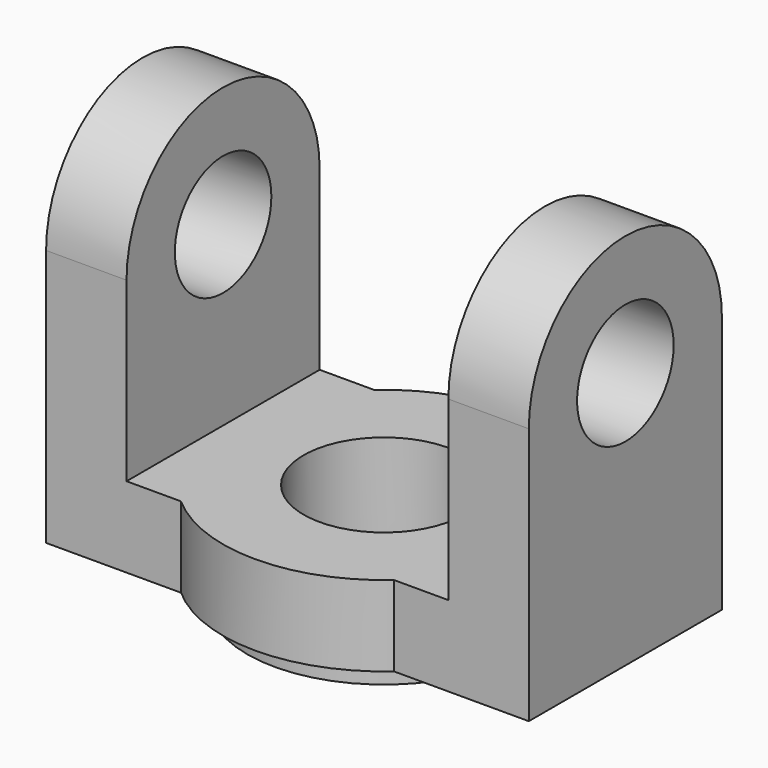
from build123d import *

# Parameters (mm, degrees)
F0_W      = 60
F0_H      = 10
F1_DEPTH  = 30
F3_DEPTH  = 3
F5_DEPTH  = 10
F6_R      = 10
F7_DEPTH  = 25
F8_R      = 10
F9_DEPTH  = 3
F10_W     = 10
F10_H     = 30
F11_DEPTH = 22
F12_R     = 15
F13_DEPTH = 10
F14_R     = 15
F15_DEPTH = 10
F16_R     = 7.5
F17_DEPTH = 60


with BuildPart() as f1:
    # F0 (on Front) → F1 (new body)
    with BuildSketch(Plane.XZ):
        with Locations((30, 5)):
            Rectangle(F0_W, F0_H)
    extrude(amount=F1_DEPTH)

    # F2 (on face) → F3 (join)
    with BuildSketch(Plane(origin=(0, 0, 0), x_dir=(1, 0, 0), z_dir=(0, 0, -1))):
        with BuildLine():
            ThreePointArc((22, 30), (13, 15), (22, 0))
            Line((22, 0), (38, 0))
            ThreePointArc((38, 0), (44.5773797371, 6.2535721577), (47, 15))
            ThreePointArc((47, 15), (44.5773797371, 23.7464278423), (38, 30))
            Line((38, 30), (22, 30))
        make_face()
        with BuildLine():
            ThreePointArc((38, 30), (30, 32), (22, 30))
            Line((22, 30), (38, 30))
        make_face()
    extrude(amount=F3_DEPTH)

    # F4 (on face) → F5 (join)
    with BuildSketch(Plane.XY.offset(10)):
        with BuildLine():
            ThreePointArc((43.2287565553, -30), (48.2287565553, -23.2287565553), (50, -15))
            ThreePointArc((50, -15), (48.2287565553, -6.7712434447), (43.2287565553, 0))
            Line((43.2287565553, 0), (16.7712434447, 0))
            ThreePointArc((16.7712434447, 0), (10, -15), (16.7712434447, -30))
            Line((16.7712434447, -30), (43.2287565553, -30))
        make_face()
        with BuildLine():
            Line((16.7712434447, 0), (43.2287565553, 0))
            ThreePointArc((43.2287565553, 0), (30, 5), (16.7712434447, 0))
        make_face()
        with BuildLine():
            ThreePointArc((16.7712434447, -30), (30, -35), (43.2287565553, -30))
            Line((43.2287565553, -30), (16.7712434447, -30))
        make_face()
    extrude(amount=-F5_DEPTH)

    # F6 (on face) → F7 (cut)
    with BuildSketch(Plane.XY.offset(10)):
        with Locations((30, -15)):
            Circle(F6_R)
    extrude(amount=-F7_DEPTH, mode=Mode.SUBTRACT)

    # F8 (on face) → F9 (join)
    with BuildSketch(Plane(origin=(0, 0, -3), x_dir=(1, 0, 0), z_dir=(0, 0, -1))):
        with BuildLine():
            ThreePointArc((38, 0), (44.5773797371, 6.2535721577), (47, 15))
            ThreePointArc((47, 15), (44.5773797371, 23.7464278423), (38, 30))
            Line((38, 30), (22, 30))
            ThreePointArc((22, 30), (13, 15), (22, 0))
            Line((22, 0), (38, 0))
        make_face()
        with Locations((30, 15)):
            Circle(F8_R, mode=Mode.SUBTRACT)
        with BuildLine():
            ThreePointArc((22, 0), (30, -2), (38, 0))
            Line((38, 0), (22, 0))
        make_face()
    extrude(amount=-F9_DEPTH)

    # F10 (on face) → F11 (join)
    with BuildSketch(Plane.XY.offset(10)):
        with Locations((5, -15)):
            Rectangle(F10_W, F10_H)
        with Locations((55, -15)):
            Rectangle(F10_W, F10_H)
    extrude(amount=F11_DEPTH)

    # F12 (on face) → F13 (join)
    with BuildSketch(Plane(origin=(0, 0, 0), x_dir=(0, -1, 0), z_dir=(-1, 0, 0))):
        with Locations((15, 32)):
            Circle(F12_R)
    extrude(amount=-F13_DEPTH)

    # F14 (on face) → F15 (join)
    with BuildSketch(Plane.YZ.offset(60)):
        with Locations((-15, 32)):
            Circle(F14_R)
    extrude(amount=-F15_DEPTH)

    # F16 (on face) → F17 (cut)
    with BuildSketch(Plane.YZ.offset(60)):
        with Locations((-15, 32)):
            Circle(F16_R)
    extrude(amount=-F17_DEPTH, mode=Mode.SUBTRACT)


solid = f1.part
